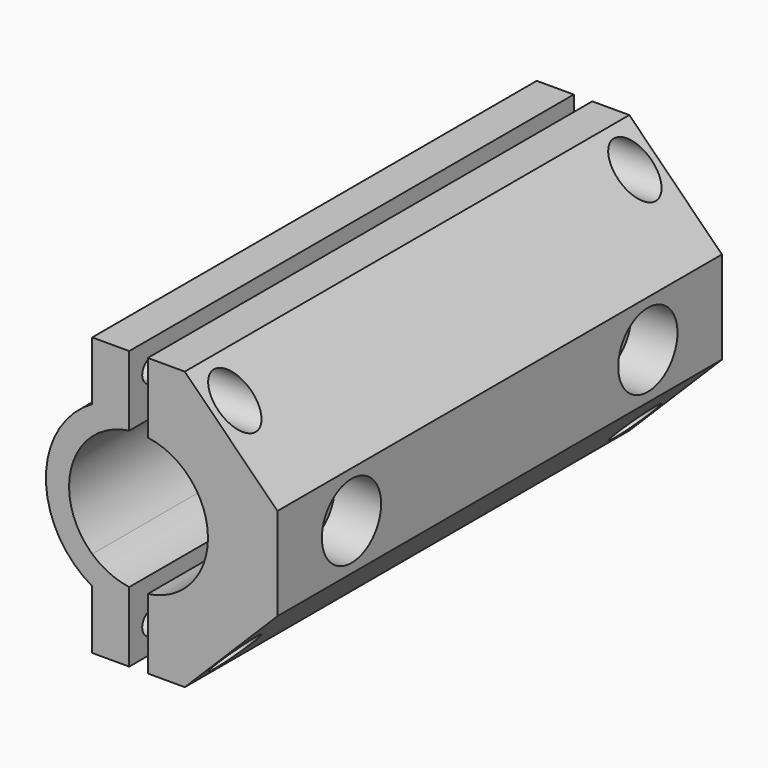
from build123d import *

# Parameters (mm, degrees)
F0_R        = 4
F1_DEPTH    = 200
F3_R        = 4
F4_DEPTH    = 5
F3_R_2      = 5
F4_FACE_R   = 5
F4_FACE_R_2 = 4
F1_FACE_R   = 4
F2_FACE_R   = 4
F3_W        = 60.0000001103
F3_H        = 30
F5_DEPTH    = 30
F7_DEPTH    = 60.0010001103
F8_DEPTH    = 60.0010001103
F9_SIZE     = 9.99999
F11_DEPTH   = 25
F13_START   = -2
F12_R       = 2.25
F12_R_2     = 1.25
F13_DEPTH   = 23
F14_DEPTH   = 200
F15_DEPTH   = 5


# Not quite as in the source:
# - a fillet or chamfer is up to 0.001 mm smaller than in the source, because OpenCascade refuses the exact size
# - a pattern or mirror of a feature is missing from the dataset's text; its kind, count and spacing are read off the source's solid
# - a feature names something its author has since deleted; it is built from what else it names


with BuildPart() as f1:
    # F0 (on Right) → F1 (new body)
    with BuildSketch(Plane.YZ):
        Circle(F0_R)
    extrude(amount=F1_DEPTH)


with BuildPart() as f2_1:
    # F2: copy of F1
    add(f1.part.moved(Location((0, -40, 0))))


with BuildPart() as f4:
    # F3 (on face) → F4 (new body)
    with BuildSketch(Plane(origin=(0, 0, 0), x_dir=(0, -1, 0), z_dir=(-1, 0, 0))):
        with Locations((40, 0)):
            Circle(F3_R)
    extrude(amount=-F4_DEPTH)


with BuildPart() as f4b:
    # F3 (on face) → F4, piece 2 (new body)
    with BuildSketch(Plane(origin=(0, 0, 0), x_dir=(0, -1, 0), z_dir=(-1, 0, 0))):
        Circle(F3_R_2)
        Circle(F3_R, mode=Mode.SUBTRACT)
    extrude(amount=-F4_DEPTH)


with BuildPart() as f1_1:
    add(f1.part)

    add(f2_1.part)  # F5 merges F2_1

    add(f4.part)  # F5 merges F4

    add(f4b.part)  # F5 merges F4b
    # F4_face (on face) + F1_face (on face) + F2_face (on face) + F3 (on face) → F5 (join)
    with BuildSketch(Plane(origin=(0, 0, 0), x_dir=(0, -1, 0), z_dir=(-1, 0, 0))):
        Circle(F4_FACE_R)
        Circle(F4_FACE_R_2, mode=Mode.SUBTRACT)
        with Locations((40, 0)):
            Circle(F4_FACE_R_2)
    with BuildSketch(Plane(origin=(0, 0, 0), x_dir=(0, 1, 0), z_dir=(-1, 0, 0))):
        Circle(F1_FACE_R)
    with BuildSketch(Plane(origin=(0, -40, 0), x_dir=(0, -1, 0), z_dir=(-1, 0, 0))):
        Circle(F2_FACE_R)
    with BuildSketch(Plane(origin=(0, 0, 0), x_dir=(0, -1, 0), z_dir=(-1, 0, 0))):
        with Locations((19.9999999448, 0)):
            Rectangle(F3_W, F3_H)
        Circle(F3_R_2, mode=Mode.SUBTRACT)
        with Locations((40, 0)):
            Circle(F3_R_2, mode=Mode.SUBTRACT)
        with Locations((40, 0)):
            Circle(F3_R_2)
        with Locations((40, 0)):
            Circle(F3_R, mode=Mode.SUBTRACT)
    extrude(amount=F5_DEPTH)

    # F6 (on face) → F7 (cut, through all)
    with BuildSketch(Plane.XZ.offset(50)):
        with BuildLine():
            Line((-10, -5.5901699437), (-10, 5.5901699437))
            ThreePointArc((-10, 5.5901699437), (-11.8616824051, 6.8118252087), (-14, 7.4330343737))
            Line((-14, 7.4330343737), (-14, -7.4330343737))
            ThreePointArc((-14, -7.4330343737), (-11.8616824051, -6.8118252087), (-10, -5.5901699437))
        make_face()
        with BuildLine():
            Line((-14, -7.4330343737), (-14, 7.4330343737))
            ThreePointArc((-14, 7.4330343737), (-15, 7.5), (-16, 7.4330343737))
            Line((-16, 7.4330343737), (-16, -7.4330343737))
            ThreePointArc((-16, -7.4330343737), (-15, -7.5), (-14, -7.4330343737))
        make_face()
        with BuildLine():
            Line((-16, -7.4330343737), (-16, 7.4330343737))
            ThreePointArc((-16, 7.4330343737), (-18.1383175949, 6.8118252087), (-20, 5.5901699437))
            Line((-20, 5.5901699437), (-20, -5.5901699437))
            ThreePointArc((-20, -5.5901699437), (-18.1383175949, -6.8118252087), (-16, -7.4330343737))
        make_face()
        with BuildLine():
            ThreePointArc((-10, -5.5901699437), (-8.1534680312, -3.0618621785), (-7.5, 0))
            ThreePointArc((-7.5, 0), (-8.1534680312, 3.0618621785), (-10, 5.5901699437))
            Line((-10, 5.5901699437), (-10, -5.5901699437))
        make_face()
        with BuildLine():
            Line((-20, -5.5901699437), (-20, 5.5901699437))
            ThreePointArc((-20, 5.5901699437), (-22.5, 0), (-20, -5.5901699437))
        make_face()
        with BuildLine():
            ThreePointArc((-16, 9.9498743711), (-15, 10), (-14, 9.9498743711))
            Line((-14, 9.9498743711), (-14, 15))
            Line((-14, 15), (-16, 15))
            Line((-16, 15), (-16, 9.9498743711))
        make_face()
        with BuildLine():
            ThreePointArc((-16, 7.4330343737), (-15, 7.5), (-14, 7.4330343737))
            Line((-14, 7.4330343737), (-14, 9.9498743711))
            ThreePointArc((-14, 9.9498743711), (-15, 10), (-16, 9.9498743711))
            Line((-16, 9.9498743711), (-16, 7.4330343737))
        make_face()
        with BuildLine():
            Line((-14, -9.9498743711), (-14, -7.4330343737))
            ThreePointArc((-14, -7.4330343737), (-15, -7.5), (-16, -7.4330343737))
            Line((-16, -7.4330343737), (-16, -9.9498743711))
            ThreePointArc((-16, -9.9498743711), (-15, -10), (-14, -9.9498743711))
        make_face()
        with BuildLine():
            Line((-14, -15), (-14, -9.9498743711))
            ThreePointArc((-14, -9.9498743711), (-15, -10), (-16, -9.9498743711))
            Line((-16, -9.9498743711), (-16, -15))
            Line((-16, -15), (-14, -15))
        make_face()
    extrude(amount=-F7_DEPTH, mode=Mode.SUBTRACT)

    # F6 (on face) → F8 (cut, through all)
    with BuildSketch(Plane.XZ.offset(50)):
        with BuildLine():
            ThreePointArc((-20, -8.6602540378), (-25, 0), (-20, 8.6602540378))
            Line((-20, 8.6602540378), (-20, 15))
            Line((-20, 15), (-30, 15))
            Line((-30, 15), (-30, -15))
            Line((-30, -15), (-20, -15))
            Line((-20, -15), (-20, -8.6602540378))
        make_face()
    extrude(amount=-F8_DEPTH, mode=Mode.SUBTRACT)

    # F9 (size 10 in the source; OpenCascade refuses exactly that, so slightly less here)
    f9_edges = [f1_1.edges().sort_by_distance(p)[0] for p in [
        (0, -20, 15),
        (0, -20, -15),
    ]]
    chamfer(f9_edges, length=F9_SIZE)

    # F10 (on face) → F11 (cut)
    with BuildSketch(Plane(origin=(-20, 0, 0), x_dir=(0, -1, 0), z_dir=(-1, 0, 0))):
        with BuildLine():
            Line((-7.0000001103, 12), (-7.0000001103, 10.75))
            ThreePointArc((-7.0000001103, 10.75), (-6.1161166338, 11.1161165235), (-5.7500001103, 12))
            Line((-5.7500001103, 12), (-7.0000001103, 12))
        make_face()
        with BuildLine():
            ThreePointArc((-5.7500001103, 12), (-7.8838835868, 12.8838834765), (-7.0000001103, 10.75))
            Line((-7.0000001103, 10.75), (-7.0000001103, 12))
            Line((-7.0000001103, 12), (-5.7500001103, 12))
        make_face()
        with BuildLine():
            ThreePointArc((45.75, 12), (46.1161165235, 11.1161165235), (47, 10.75))
            Line((47, 10.75), (47, 12))
            Line((47, 12), (45.75, 12))
        make_face()
        with BuildLine():
            Line((47, 12), (47, 10.75))
            ThreePointArc((47, 10.75), (47.8838834765, 11.1161165235), (48.25, 12))
            ThreePointArc((48.25, 12), (47, 13.25), (45.75, 12))
            Line((45.75, 12), (47, 12))
        make_face()
        with BuildLine():
            ThreePointArc((47, -10.75), (46.1161165235, -11.1161165235), (45.75, -12))
            Line((45.75, -12), (47, -12))
            Line((47, -12), (47, -10.75))
        make_face()
        with BuildLine():
            Line((47, -12), (45.75, -12))
            ThreePointArc((45.75, -12), (47, -13.25), (48.25, -12))
            ThreePointArc((48.25, -12), (47.8838834765, -11.1161165235), (47, -10.75))
            Line((47, -10.75), (47, -12))
        make_face()
        with BuildLine():
            ThreePointArc((-5.7500001103, -12), (-6.1161166338, -11.1161165235), (-7.0000001103, -10.75))
            Line((-7.0000001103, -10.75), (-7.0000001103, -12))
            Line((-7.0000001103, -12), (-5.7500001103, -12))
        make_face()
        with BuildLine():
            Line((-7.0000001103, -12), (-7.0000001103, -10.75))
            ThreePointArc((-7.0000001103, -10.75), (-7.8838835868, -12.8838834765), (-5.7500001103, -12))
            Line((-5.7500001103, -12), (-7.0000001103, -12))
        make_face()
    extrude(amount=-F11_DEPTH, mode=Mode.SUBTRACT)

    # F12 (on face) → F13 (cut)
    with BuildSketch(Plane(origin=(-14, 0, 0), x_dir=(0, -1, 0), z_dir=(-1, 0, 0)).offset(F13_START)):
        with Locations((47, 12)):
            Circle(F12_R)
        with Locations((47, 12)):
            Circle(F12_R_2, mode=Mode.SUBTRACT)
        with Locations((47, -12)):
            Circle(F12_R)
        with Locations((-7.0000001103, -12)):
            Circle(F12_R)
        with Locations((-7.0000001103, 12)):
            Circle(F12_R)
        with Locations((-7.0000001103, 12)):
            Circle(F12_R_2, mode=Mode.SUBTRACT)
    extrude(amount=-F13_DEPTH, mode=Mode.SUBTRACT)

    # F14 (cut, through all): faces of the model
    f14_faces = [f1_1.faces().sort_by_distance(p)[0] for p in [
        (200, -40, 0),
        (200, 0, 0),
    ]]
    extrude(f14_faces, amount=-F14_DEPTH, mode=Mode.SUBTRACT)

    # F15 (cut): faces of the model
    f15_faces = [f1_1.faces().sort_by_distance(p)[0] for p in [
        (0, 0, 0),
        (0, 0, 0),
        (5, 4.8585786438, 0),
    ]]
    f15 = extrude(f15_faces, amount=-F15_DEPTH, mode=Mode.SUBTRACT)

    # F15_copies: F15 across plane
    add(f15.mirror(Plane(origin=(0, -20, 0), x_dir=(0, 0, -1), z_dir=(0, -1, 0))), mode=Mode.SUBTRACT)


solid = f1_1.part
